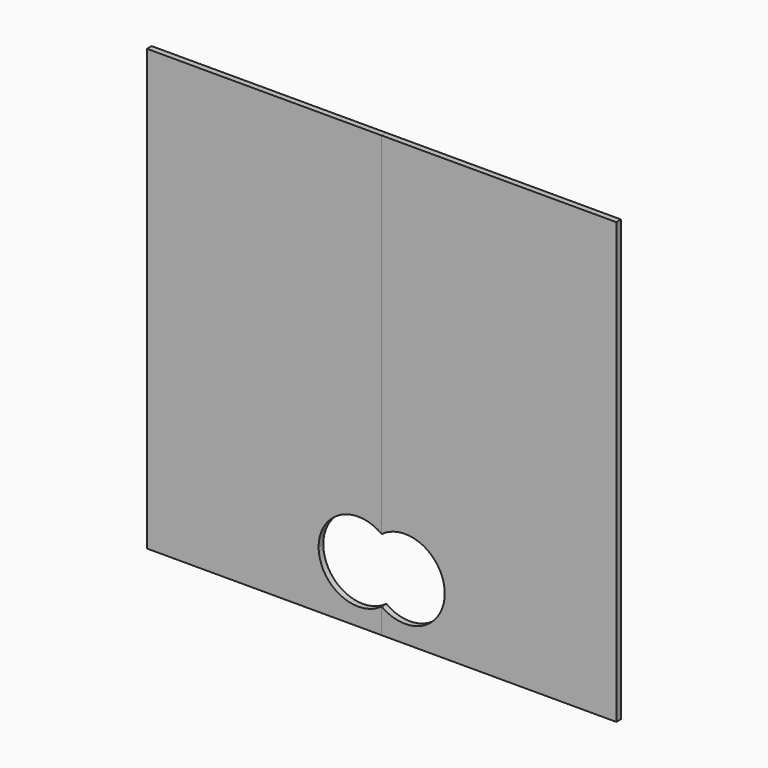
from build123d import *

# Parameters (mm, degrees)
F1_DEPTH = 2


# Not quite as in the source:
# - a feature names something its author has since deleted; it is built from what else it names


with BuildPart() as f1:
    # F0 (on Front) → F1 (new body)
    with BuildSketch(Plane.XZ):
        with BuildLine():
            Line((0, 0), (80, 0))
            Line((80, 0), (80, 150))
            Line((80, 150), (0, 150))
            Line((0, 150), (0, 30.3742815855))
            ThreePointArc((0, 30.3742815855), (14.0930288035, 31.5467838032), (21.5, 19.5))
            ThreePointArc((21.5, 19.5), (14.0930288035, 7.4532161968), (0, 8.6257184145))
            Line((0, 8.6257184145), (0, 0))
        make_face()
    extrude(amount=-F1_DEPTH)


with BuildPart() as f2_1:
    # F2: instance of F1
    add(f1.part.mirror(Plane.YZ))


solid = Compound([f1.part, f2_1.part])
